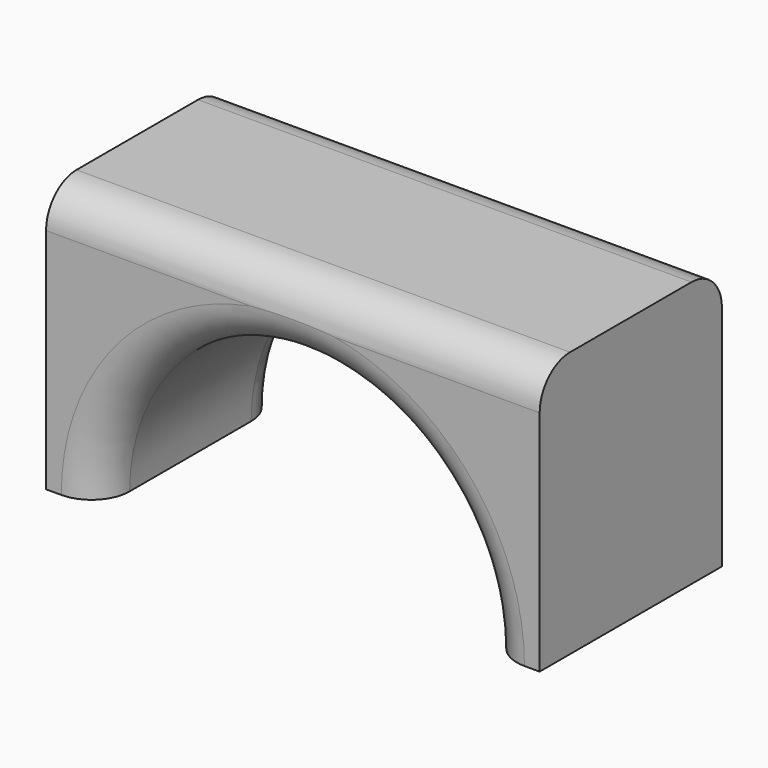
from build123d import *

# Parameters (mm, degrees)
F1_DEPTH    = 30
F2_T1_DEPTH = 90
F2_T4_ANGLE = 236.2626685885
F2_T6_ANGLE = 236.2626685885


# Not quite as in the source:
# - a fillet or chamfer that OpenCascade refuses, or shapes differently, is made with other operations: its cross-section is extruded or revolved along the edge and cut away or added


with BuildPart() as f1:
    # F0 (on Front) → F1 (new body)
    with BuildSketch(Plane.XZ):
        with BuildLine():
            Line((0, 35), (0, 0))
            Line((0, 0), (7, 0))
            ThreePointArc((7, 0), (32.5, 25.5), (58, 0))
            Line((58, 0), (65, 0))
            Line((65, 0), (65, 35))
            Line((65, 35), (0, 35))
        make_face()
    extrude(amount=F1_DEPTH)

    # F2: fillet of radius 5 on 4 edges, made by hand

    # F2_s2 → F2_t1 (cut)
    with BuildSketch(Plane.YZ.offset(-12.5)):
        with BuildLine():
            ThreePointArc((-25, 35), (-28.5355339059, 33.5355339059), (-30, 30))
            Line((-30, 30), (-30, 35))
            Line((-30, 35), (-25, 35))
        make_face()
        with BuildLine():
            ThreePointArc((-5, 35), (-1.4644660941, 33.5355339059), (0, 30))
            Line((0, 30), (0, 35))
            Line((0, 35), (-5, 35))
        make_face()
    extrude(amount=F2_T1_DEPTH, mode=Mode.SUBTRACT)

    # F2_s3 → F2_t4 (revolve, cut)
    with BuildSketch(Plane(origin=(7.2249714164, 0, -13.5133770415), x_dir=(0, 1, 0), z_dir=(0.4714942341, 0, -0.881869144))):
        with BuildLine():
            ThreePointArc((-25, 3.1607471809), (-28.5355339059, 1.6962810868), (-30, -1.8392528191))
            Line((-30, -1.8392528191), (-30, 3.1607471809))
            Line((-30, 3.1607471809), (-25, 3.1607471809))
        make_face()
    revolve(axis=Axis((32.5, -30, 0), (0, 1, 0)), revolution_arc=F2_T4_ANGLE, mode=Mode.SUBTRACT)

    # F2_s5 → F2_t6 (revolve, cut)
    with BuildSketch(Plane(origin=(7.2249714164, 0, -13.5133770415), x_dir=(0, 1, 0), z_dir=(0.4714942341, 0, -0.881869144))):
        with BuildLine():
            ThreePointArc((-5, 3.1607471809), (-1.4644660941, 1.6962810868), (0, -1.8392528191))
            Line((0, -1.8392528191), (0, 3.1607471809))
            Line((0, 3.1607471809), (-5, 3.1607471809))
        make_face()
    revolve(axis=Axis((32.5, 0, 0), (0, 1, 0)), revolution_arc=F2_T6_ANGLE, mode=Mode.SUBTRACT)


solid = f1.part
